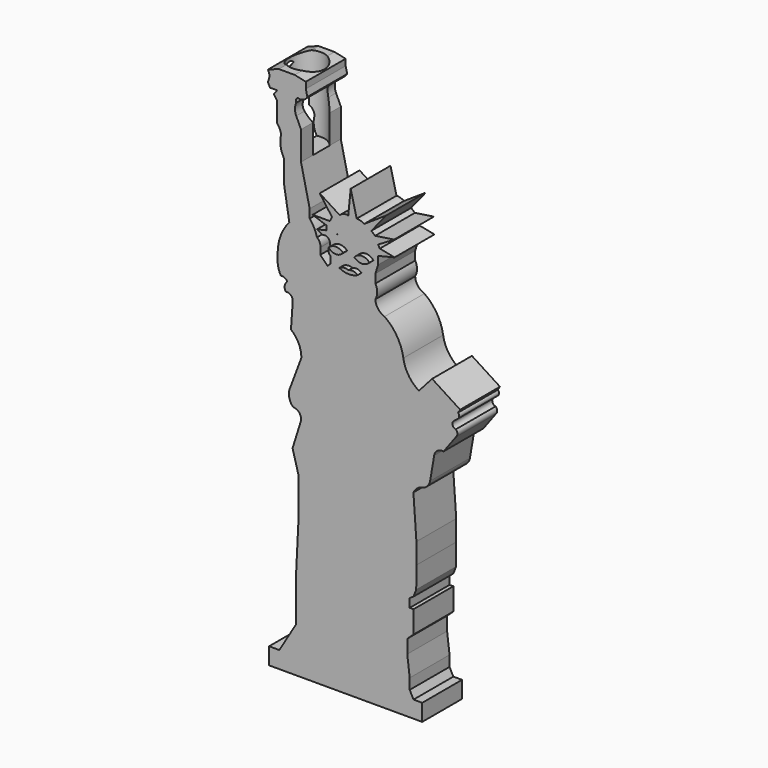
from build123d import *

# Parameters (mm, degrees)
F1_DEPTH = 12.7
F5_DEPTH = 1.27
F7_DEPTH = 13.97
F8_R     = 4.5
F9_DEPTH = 19.05


# Not quite as in the source:
# - the program builds the solid bodies; features that only make, move or delete a surface that nothing else refers to are left out


with BuildPart() as f1:
    # F0 (on Front) → F1 (new body)
    with BuildSketch(Plane.XZ):
        with BuildLine():
            Line((-24.262432009, -66.7880773544), (-24.262432009, -71.0822939873))
            Line((-24.262432009, -71.0822939873), (14.8010868579, -71.0822939873))
            Line((14.8010868579, -71.0822939873), (14.8010868579, -66.7880773544))
            Line((14.8010868579, -66.7880773544), (12.5847170129, -66.7880773544))
            Line((12.5847170129, -66.7880773544), (11.6150556132, -64.9180188775))
            Line((11.6150556132, -64.9180188775), (11.6150556132, -62.2168146074))
            Line((11.6150556132, -62.2168146074), (10.9917018563, -57.0914596319))
            Line((10.9917018563, -57.0914596319), (10.9917018563, -53.6283813417))
            Line((10.9917018563, -53.6283813417), (12.5847170129, -52.1738901734))
            Line((12.5847170129, -52.1738901734), (12.5847170129, -46.4944429696))
            Line((12.5847170129, -46.4944429696), (11.6150556132, -46.4944429696))
            Line((11.6150556132, -46.4944429696), (11.6150556132, -44.2780740559))
            Line((11.6150556132, -44.2780740559), (12.5847170129, -43.654717505))
            Line((12.5847170129, -43.654717505), (13.2773322985, -41.8539159))
            Line((13.2773322985, -41.8539159), (13.3222565055, -36.3315418363))
            Line((13.3222565055, -36.3315418363), (13.3222565055, -31.0600940138))
            Line((13.3222565055, -31.0600940138), (12.5571293756, -20.2698614448))
            ThreePointArc((12.5571293756, -20.2698614448), (13.3767429513, -19.1417378809), (14.5955923945, -18.4643641114))
            ThreePointArc((14.5955923945, -18.4643641114), (16.0561590622, -17.7622935329), (16.8151462827, -16.3304777322))
            Line((16.8151462827, -16.3304777322), (17.8571324795, -10.2522717789))
            ThreePointArc((17.8571324795, -10.2522717789), (18.7012837928, -8.913213743), (20.2450454235, -8.5632596165))
            Line((20.2450454235, -8.5632596165), (23.3847144991, -4.3181492947))
            ThreePointArc((23.3847144991, -4.3181492947), (23.7706037969, -3.4445220372), (23.3847144991, -2.5708947796))
            ThreePointArc((23.3847144991, -2.5708947796), (22.5482496559, -1.8772318765), (22.873915941, -0.8405143991))
            Line((22.873915941, -0.8405143991), (23.923975447, 0))
            ThreePointArc((23.923975447, 0), (24.2414660644, 0.6608081876), (23.923975447, 1.3216163752))
            Line((23.923975447, 1.3216163752), (24.491308257, 2.2049320396))
            Line((24.491308257, 2.2049320396), (17.3275675625, 6.8060336635))
            Line((17.3275675625, 6.8060336635), (13.9495451003, 3.0203172937))
            ThreePointArc((13.9495451003, 3.0203172937), (11.3103546035, 5.6180262749), (9.989102371, 9.0774642304))
            ThreePointArc((9.989102371, 9.0774642304), (8.3833020972, 13.444705978), (5.2074426785, 16.8454870582))
            ThreePointArc((5.2074426785, 16.8454870582), (3.5424271588, 18.0354865682), (2.8525488451, 19.9622567743))
            ThreePointArc((2.8525488451, 19.9622567743), (3.3166855473, 21.728426218), (2.8525488451, 23.4945956618))
            Line((2.8525488451, 23.4945956618), (2.8525488451, 25.7109664381))
            Line((2.8525488451, 25.7109664381), (3.5320665038, 27.9273353517))
            Line((3.5320665038, 27.9273353517), (3.5320665038, 29.935920611))
            ThreePointArc((3.5320665038, 29.935920611), (3.1612311526, 30.2705017109), (2.7725197573, 30.5841365643))
            ThreePointArc((2.7725197573, 30.5841365643), (2.0633515274, 31.0732427581), (1.3109308964, 31.4927754042))
            ThreePointArc((1.3109308964, 31.4927754042), (0.6657809293, 31.7824572219), (0, 32.0209310982))
            ThreePointArc((0, 32.0209310982), (-2.1735489756, 32.4223132924), (-4.3796033975, 32.2853946937))
            ThreePointArc((-4.3796033975, 32.2853946937), (-4.9757005258, 32.1533551463), (-5.5615500383, 31.981463968))
            ThreePointArc((-5.5615500383, 31.981463968), (-5.9334399833, 31.8495443963), (-6.2992323982, 31.7015551605))
            Line((-6.2992323982, 31.7015551605), (-6.9038875562, 31.3904136419))
            Line((-6.9038875562, 31.3904136419), (-7.4102797015, 31.1298359903))
            ThreePointArc((-7.4102797015, 31.1298359903), (-7.8425965144, 30.8511130482), (-8.2583969346, 30.5483023554))
            ThreePointArc((-8.2583969346, 30.5483023554), (-8.7062340241, 30.1787716739), (-9.1294797515, 29.7813121949))
            ThreePointArc((-9.1294797515, 29.7813121949), (-8.9029048756, 29.4703282829), (-8.7822196609, 29.1049760598))
            Line((-8.7822196609, 29.1049760598), (-8.6448690854, 28.2736439258))
            ThreePointArc((-8.6448690854, 28.2736439258), (-9.1392904513, 27.130828239), (-8.6448690854, 25.9880125523))
            Line((-8.6448690854, 25.9880125523), (-8.6448690854, 24.1872114129))
            Line((-8.6448690854, 24.1872114129), (-9.3374848366, 23.4945956618))
            Line((-9.3374848366, 23.4945956618), (-11.2075470388, 25.364657864))
            Line((-11.2075470388, 25.364657864), (-11.2075470388, 27.0269364119))
            ThreePointArc((-11.2075470388, 27.0269364119), (-11.3449435763, 28.1463349056), (-12.0386853814, 29.0355216712))
            ThreePointArc((-12.0386853814, 29.0355216712), (-12.7642988711, 30.9450584102), (-13.9087475836, 32.6371230185))
            Line((-13.9087475836, 32.6371230185), (-13.9087475836, 34.8534919322))
            Line((-13.9087475836, 34.8534919322), (-16.1189688019, 44.6193702519))
            Line((-16.1189688019, 44.6193702519), (-16.1189688019, 48.955809325))
            Line((-16.1189688019, 48.955809325), (-16.1189688019, 51.9356569561))
            Line((-16.1189688019, 51.9356569561), (-17.3431094736, 54.5879676938))
            ThreePointArc((-17.3431094736, 54.5879676938), (-17.6658124636, 56.0572277755), (-17.3431094736, 57.5264878571))
            ThreePointArc((-17.3431094736, 57.5264878571), (-17.4062332067, 58.2407443521), (-16.9023312628, 58.7508715689))
            ThreePointArc((-16.9023312628, 58.7508715689), (-15.5109918355, 58.8184091315), (-14.5025411621, 59.7793534398))
            Line((-14.5025411621, 59.7793534398), (-14.8943439126, 61.4445134997))
            Line((-14.8943439126, 61.4445134997), (-14.8943439126, 63.0607008934))
            Line((-14.8943439126, 63.0607008934), (-17.7349131554, 63.6684481159))
            Line((-17.7349131554, 63.6684481159), (-21.7659391535, 63.6684481159))
            Line((-21.7659391535, 63.6684481159), (-24.5424807072, 62.6688972116))
            Line((-24.5424807072, 62.6688972116), (-24.1017043591, 61.4445134997))
            Line((-24.1017043591, 61.4445134997), (-24.5424807072, 59.8283298314))
            Line((-24.5424807072, 59.8283298314), (-24.0527279675, 58.7508715689))
            Line((-24.0527279675, 58.7508715689), (-22.2088433802, 58.7508715689))
            Line((-22.2088433802, 58.7508715689), (-23.0732224882, 57.6734133065))
            Line((-23.0732224882, 57.6734133065), (-22.2088433802, 56.3510805368))
            Line((-22.2088433802, 56.3510805368), (-22.2088433802, 51.3100810349))
            ThreePointArc((-22.2088433802, 51.3100810349), (-21.5097946529, 50.2632850834), (-21.218733862, 49.0386486053))
            ThreePointArc((-21.218733862, 49.0386486053), (-21.318722088, 46.4228178095), (-20.4243380576, 43.9626052976))
            Line((-20.4243380576, 43.9626052976), (-20.4243380576, 38.0753725767))
            Line((-20.4243380576, 38.0753725767), (-19.1083680838, 30.1102939993))
            ThreePointArc((-19.1083680838, 30.1102939993), (-21.3102077241, 26.4315508709), (-22.0875215801, 22.2152690996))
            Line((-22.0875215801, 22.2152690996), (-22.093527019, 20.635003224))
            ThreePointArc((-22.093527019, 20.635003224), (-21.8856045583, 18.9543406711), (-21.2623886764, 17.3797104508))
            ThreePointArc((-21.2623886764, 17.3797104508), (-20.3211034807, 17.3053690653), (-19.6317378432, 16.6601408273))
            ThreePointArc((-19.6317378432, 16.6601408273), (-20.2775112214, 15.5197902404), (-20.0435705483, 14.2303351313))
            ThreePointArc((-20.0435705483, 14.2303351313), (-18.7459820263, 13.9012384012), (-18.231511116, 12.6653742045))
            Line((-18.231511116, 12.6653742045), (-18.6845250428, 6.1584338546))
            ThreePointArc((-18.6845250428, 6.1584338546), (-16.7243053359, 3.7123480406), (-16.0280633718, 0.6560358452))
            Line((-16.0280633718, 0.6560358452), (-19.0645344555, -7.4248914607))
            ThreePointArc((-19.0645344555, -7.4248914607), (-19.0881113009, -9.385305908), (-18.1340035051, -11.0980402678))
            ThreePointArc((-18.1340035051, -11.0980402678), (-16.5009554932, -11.9102931717), (-16.196295619, -13.7085653841))
            Line((-16.196295619, -13.7085653841), (-18.2741414756, -20.3576739877))
            Line((-18.2741414756, -20.3576739877), (-16.7503878474, -25.9678605944))
            Line((-16.7503878474, -25.9678605944), (-16.7503878474, -35.595215857))
            Line((-16.7503878474, -35.595215857), (-17.4443386495, -49.6193654835))
            Line((-17.4443386495, -49.6193654835), (-17.4443386495, -59.7221441567))
            Line((-17.4443386495, -59.7221441567), (-21.6377470642, -66.7880773544))
            Line((-21.6377470642, -66.7880773544), (-24.262432009, -66.7880773544))
        make_face()
        with BuildLine():
            ThreePointArc((3.9826073295, 31.7208051674), (4.1270140297, 30.7350489373), (3.5320665038, 29.935920611))
            Line((3.5320665038, 29.935920611), (7.7701197006, 30.9748444706))
            Line((7.7701197006, 30.9748444706), (3.9826073295, 31.7208051674))
        make_face()
        with BuildLine():
            ThreePointArc((2.7725197573, 30.5841365643), (3.1612311526, 30.2705017109), (3.5320665038, 29.935920611))
            ThreePointArc((3.5320665038, 29.935920611), (4.1270140297, 30.7350489373), (3.9826073295, 31.7208051674))
            Line((3.9826073295, 31.7208051674), (2.7725197573, 30.5841365643))
        make_face()
        with BuildLine():
            ThreePointArc((1.3109308964, 31.4927754042), (2.0633515274, 31.0732427581), (2.7725197573, 30.5841365643))
            Line((2.7725197573, 30.5841365643), (3.9826073295, 31.7208051674))
            Line((3.9826073295, 31.7208051674), (3.5320665038, 32.4755454095))
            ThreePointArc((3.5320665038, 32.4755454095), (3.096905621, 33.2448661733), (2.6982102432, 34.0337016614))
            Line((2.6982102432, 34.0337016614), (1.3109308964, 31.4927754042))
        make_face()
        with BuildLine():
            ThreePointArc((0, 32.0209310982), (0.6657809293, 31.7824572219), (1.3109308964, 31.4927754042))
            Line((1.3109308964, 31.4927754042), (2.6982102432, 34.0337016614))
            Line((2.6982102432, 34.0337016614), (2.7912367903, 34.2040881065))
            Line((2.7912367903, 34.2040881065), (1.813625684, 34.9920131266))
            ThreePointArc((1.813625684, 34.9920131266), (0.9523713324, 35.5620558321), (0, 35.961676389))
            Line((0, 35.961676389), (0, 32.0209310982))
        make_face()
        with BuildLine():
            ThreePointArc((2.6982102432, 34.0337016614), (3.096905621, 33.2448661733), (3.5320665038, 32.4755454095))
            Line((3.5320665038, 32.4755454095), (7.6315966435, 34.9227525294))
            Line((7.6315966435, 34.9227525294), (2.7912367903, 34.2040881065))
            Line((2.7912367903, 34.2040881065), (2.6982102432, 34.0337016614))
        make_face()
        with BuildLine():
            ThreePointArc((-4.3796033975, 32.2853946937), (-2.1735489756, 32.4223132924), (0, 32.0209310982))
            Line((0, 32.0209310982), (0, 35.961676389))
            ThreePointArc((0, 35.961676389), (-0.9208363251, 36.3861856607), (-1.9264982548, 36.5157686174))
            ThreePointArc((-1.9264982548, 36.5157686174), (-3.0000525294, 36.577229853), (-4.073606804, 36.5157686174))
            ThreePointArc((-4.073606804, 36.5157686174), (-4.3710717678, 36.5841594986), (-4.6754318785, 36.6071299207))
            Line((-4.6754318785, 36.6071299207), (-4.3796033975, 32.2853946937))
        make_face()
        with BuildLine():
            ThreePointArc((-5.5615500383, 31.981463968), (-4.9757005258, 32.1533551463), (-4.3796033975, 32.2853946937))
            Line((-4.3796033975, 32.2853946937), (-4.6754318785, 36.6071299207))
            ThreePointArc((-4.6754318785, 36.6071299207), (-5.5267125527, 36.4197987859), (-6.2207146548, 35.8924157917))
            Line((-6.2207146548, 35.8924157917), (-6.9220978767, 35.0996181369))
            Line((-6.9220978767, 35.0996181369), (-5.5615500383, 31.981463968))
        make_face()
        with BuildLine():
            Line((5.5537503213, 39.6325401962), (0, 35.961676389))
            ThreePointArc((0, 35.961676389), (0.9523713324, 35.5620558321), (1.813625684, 34.9920131266))
            Line((1.813625684, 34.9920131266), (5.5537503213, 39.6325401962))
        make_face()
        with BuildLine():
            ThreePointArc((-6.2992323982, 31.7015551605), (-5.9334399833, 31.8495443963), (-5.5615500383, 31.981463968))
            Line((-5.5615500383, 31.981463968), (-6.9220978767, 35.0996181369))
            Line((-6.9220978767, 35.0996181369), (-8.197018071, 34.8171565511))
            Line((-8.197018071, 34.8171565511), (-8.7822196609, 33.7453074753))
            Line((-8.7822196609, 33.7453074753), (-6.9174807235, 31.4074556047))
            ThreePointArc((-6.9174807235, 31.4074556047), (-6.6111358391, 31.560347908), (-6.2992323982, 31.7015551605))
        make_face()
        with BuildLine():
            ThreePointArc((-4.073606804, 36.5157686174), (-3.0000525294, 36.577229853), (-1.9264982548, 36.5157686174))
            Line((-1.9264982548, 36.5157686174), (-3.4502528142, 42.7493080497))
            Line((-3.4502528142, 42.7493080497), (-4.073606804, 36.5157686174))
        make_face()
        Polygon((-8.197018071, 34.8171565511), (-6.9220978767, 35.0996181369), (-6.2207146548, 35.8924157917), (-11.3460700959, 39.147708565), align=None)
        with BuildLine():
            ThreePointArc((-7.4102797015, 31.1298359903), (-7.166047429, 31.2724927954), (-6.9174807235, 31.4074556047))
            Line((-6.9174807235, 31.4074556047), (-8.7822196609, 33.7453074753))
            ThreePointArc((-8.7822196609, 33.7453074753), (-9.1706470222, 33.1034412045), (-9.6145309508, 32.4985980988))
            Line((-9.6145309508, 32.4985980988), (-9.6145309508, 31.3904136419))
            Line((-9.6145309508, 31.3904136419), (-8.2583969346, 30.5483023554))
            ThreePointArc((-8.2583969346, 30.5483023554), (-7.8425965144, 30.8511130482), (-7.4102797015, 31.1298359903))
        make_face()
        with BuildLine():
            ThreePointArc((-9.6145309508, 32.4985980988), (-9.1706470222, 33.1034412045), (-8.7822196609, 33.7453074753))
            Line((-8.7822196609, 33.7453074753), (-13.1468707696, 33.7453074753))
            Line((-13.1468707696, 33.7453074753), (-9.6145309508, 32.4985980988))
        make_face()
        with BuildLine():
            ThreePointArc((-9.1294797515, 29.7813121949), (-8.7062340241, 30.1787716739), (-8.2583969346, 30.5483023554))
            Line((-8.2583969346, 30.5483023554), (-9.6145309508, 31.3904136419))
            Line((-9.6145309508, 31.3904136419), (-12.0386853814, 30.8363214135))
            Line((-12.0386853814, 30.8363214135), (-10.5841932818, 30.0051830709))
            ThreePointArc((-10.5841932818, 30.0051830709), (-9.8201672461, 30.1315246477), (-9.1294797515, 29.7813121949))
        make_face()
    extrude(amount=F1_DEPTH)

    # F4 (on face) → F5 (join)
    with BuildSketch(Plane.XZ.offset(12.7)):
        with BuildLine():
            Line((-0.6827876205, 24.7429776937), (-5.345268175, 24.8755607754))
            ThreePointArc((-5.345268175, 24.8755607754), (-3.0301783552, 24.2413144626), (-0.6827876205, 24.7429776937))
        make_face()
        with BuildLine():
            ThreePointArc((-2.9808820691, 25.1186285168), (-4.1921091409, 25.2795164533), (-5.345268175, 24.8755607754))
            Line((-5.345268175, 24.8755607754), (-0.6827876205, 24.7429776937))
            ThreePointArc((-0.6827876205, 24.7429776937), (-1.7749657962, 25.2787071609), (-2.9808820691, 25.1186285168))
        make_face()
    extrude(amount=F5_DEPTH)

    # F6 (on Front) → F7 (join)
    with BuildSketch(Plane.XZ):
        with BuildLine():
            ThreePointArc((-1.4919285895, 28.5084210336), (0.4401657071, 27.6910023429), (2.3529604077, 28.5526160151))
            ThreePointArc((2.3529604077, 28.5526160151), (0.4200778218, 29.4386145487), (-1.4919285895, 28.5084210336))
        make_face()
        with BuildLine():
            ThreePointArc((-8.0326590687, 28.5526160151), (-6.2096514739, 27.6461715891), (-4.3866438791, 28.5526160151))
            ThreePointArc((-4.3866438791, 28.5526160151), (-6.2096514739, 29.3493131767), (-8.0326590687, 28.5526160151))
        make_face()
    extrude(amount=F7_DEPTH)

    # F8 (on face) → F9 (cut)
    with BuildSketch(Plane.XY.offset(63.6684481159)):
        with Locations((-19.7678878903, -6.2626684085)):
            Circle(F8_R)
    extrude(amount=-F9_DEPTH, mode=Mode.SUBTRACT)


solid = f1.part
